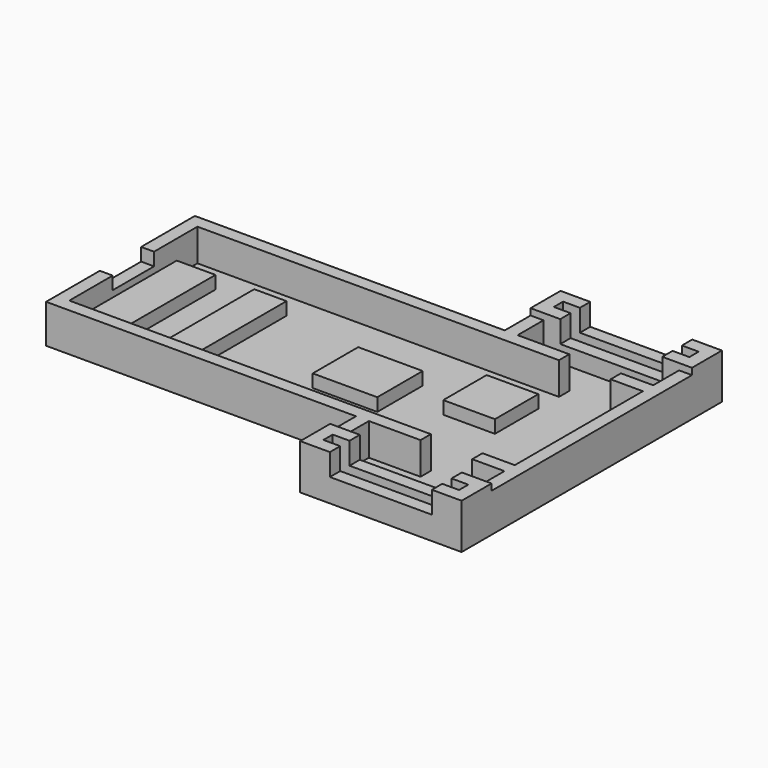
from build123d import *

# Parameters (mm, degrees)
F0_W      = 6
F0_H      = 16.8
F1_DEPTH  = 3
F0_W_2    = 5
F0_W_3    = 10
F0_H_2    = 8.8
F0_W_4    = 8
F0_H_3    = 8.4
F2_DEPTH  = 6
F0_W_5    = 15.8
F0_H_4    = 2
F3_DEPTH  = 3.6
F4_DEPTH  = 1
F7_DEPTH  = 1
F8_DEPTH  = 1
F9_W      = 2
F9_H      = 8
F10_DEPTH = 2


# Not quite as in the source:
# - a feature names something its author has since deleted; it is built from what else it names


with BuildPart() as f1:
    # F0 (on Top) → F1 (new body)
    with BuildSketch(Plane.XY):
        with Locations((3, 12.4)):
            Rectangle(F0_W, F0_H)
    extrude(amount=F1_DEPTH)

    # F0 (on Top) → F2 (join)
    with BuildSketch(Plane.XY):
        Polygon((0, 4), (0, 20.8), (0, 24.8), (56, 24.8), (56, 26.8), (48, 26.8), (48, 31.8), (50.6, 31.8), (50.6, 33.8), (48, 33.8), (48, 35.6), (50.6, 35.6), (50.6, 37.6), (46, 37.6), (46, 26.8), (-2, 26.8), (-2, -2), (46, -2), (46, -12.8), (50.6, -12.8), (50.6, -10.8), (48, -10.8), (48, -9), (50.6, -9), (50.6, -7), (48, -7), (48, -2), (56, -2), (56, 0), (0, 0), align=None)
    extrude(amount=F2_DEPTH)



with BuildPart() as f1b:
    # F0 (on Top) → F1, piece 2 (new body)
    with BuildSketch(Plane.XY):
        with Locations((14.5, 12.4)):
            Rectangle(F0_W_2, F0_H)
    extrude(amount=F1_DEPTH)


with BuildPart() as f1c:
    # F0 (on Top) → F1, piece 3 (new body)
    with BuildSketch(Plane.XY):
        with Locations((36.3, 12.4)):
            Rectangle(F0_W_3, F0_H_2)
    extrude(amount=F1_DEPTH)


with BuildPart() as f1d:
    # F0 (on Top) → F1, piece 4 (new body)
    with BuildSketch(Plane.XY):
        with Locations((52, 16.6)):
            Rectangle(F0_W_4, F0_H_3)
    extrude(amount=F1_DEPTH)


with BuildPart() as f2:
    # F0 (on Top) → F2, piece 2 (new body)
    with BuildSketch(Plane.XY):
        Polygon((66.4, 33.8), (66.4, 31.8), (69, 31.8), (69, 26.8), (64, 26.8), (64, 24.8), (69, 24.8), (69, 0), (64, 0), (64, -2), (69, -2), (69, -7), (66.4, -7), (66.4, -9), (69, -9), (69, -10.8), (66.4, -10.8), (66.4, -12.8), (71, -12.8), (71, 37.6), (66.4, 37.6), (66.4, 35.6), (69, 35.6), (69, 33.8), align=None)
    extrude(amount=F2_DEPTH)


with BuildPart() as f1_1:
    add(f1.part)

    add(f2.part)  # F3 merges F2
    # F0 (on Top) → F3 (join)
    with BuildSketch(Plane.XY):
        with Locations((58.5, 36.6)):
            Rectangle(F0_W_5, F0_H_4)
        with Locations((58.5, 32.8)):
            Rectangle(F0_W_5, F0_H_4)
        with Locations((58.5, -8)):
            Rectangle(F0_W_5, F0_H_4)
        with Locations((58.5, -11.8)):
            Rectangle(F0_W_5, F0_H_4)
    extrude(amount=F3_DEPTH)

    # F0 (on Top) → F4 (join)
    with BuildSketch(Plane.XY):
        Polygon((48, 33.8), (50.6, 33.8), (66.4, 33.8), (69, 33.8), (69, 35.6), (66.4, 35.6), (50.6, 35.6), (48, 35.6), align=None)
        Polygon((66.4, -9), (50.6, -9), (48, -9), (48, -10.8), (50.6, -10.8), (66.4, -10.8), (69, -10.8), (69, -9), align=None)
    extrude(amount=F4_DEPTH)

    # F5 (on face) + F6 (on face) → F7 (join)
    with BuildSketch(Plane.XY.offset(6)):
        Polygon((48, 31.8), (50.6, 31.8), (50.6, 33.8), (48, 33.8), (48, 35.6), (50.6, 35.6), (50.6, 37.6), (46, 37.6), (46, 31.8), align=None)
        Polygon((48, -7), (46, -7), (46, -12.8), (50.6, -12.8), (50.6, -10.8), (48, -10.8), (48, -9), (50.6, -9), (50.6, -7), align=None)
    with BuildSketch(Plane.XY.offset(6)):
        Polygon((66.4, 33.8), (66.4, 31.8), (69, 31.8), (71, 31.8), (71, 37.6), (66.4, 37.6), (66.4, 35.6), (69, 35.6), (69, 33.8), align=None)
        Polygon((71, -12.8), (71, -7), (69, -7), (66.4, -7), (66.4, -9), (69, -9), (69, -10.8), (66.4, -10.8), (66.4, -12.8), align=None)
    extrude(amount=F7_DEPTH)


    add(f1b.part)  # F8 merges F1b

    add(f1c.part)  # F8 merges F1c

    add(f1d.part)  # F8 merges F1d
    # F0 (on Top) → F8 (join)
    with BuildSketch(Plane.XY):
        Polygon((0, 4), (0, 20.8), (0, 24.8), (56, 24.8), (56, 26.8), (48, 26.8), (48, 31.8), (50.6, 31.8), (50.6, 33.8), (48, 33.8), (48, 35.6), (50.6, 35.6), (50.6, 37.6), (46, 37.6), (46, 26.8), (-2, 26.8), (-2, -2), (46, -2), (46, -12.8), (50.6, -12.8), (50.6, -10.8), (48, -10.8), (48, -9), (50.6, -9), (50.6, -7), (48, -7), (48, -2), (56, -2), (56, 0), (0, 0), align=None)
        Polygon((66.4, 33.8), (66.4, 31.8), (69, 31.8), (69, 26.8), (64, 26.8), (64, 24.8), (69, 24.8), (69, 0), (64, 0), (64, -2), (69, -2), (69, -7), (66.4, -7), (66.4, -9), (69, -9), (69, -10.8), (66.4, -10.8), (66.4, -12.8), (71, -12.8), (71, 37.6), (66.4, 37.6), (66.4, 35.6), (69, 35.6), (69, 33.8), align=None)
        with Locations((58.5, 36.6)):
            Rectangle(F0_W_5, F0_H_4)
        with Locations((58.5, -11.8)):
            Rectangle(F0_W_5, F0_H_4)
        Polygon((0, 24.8), (0, 20.8), (6, 20.8), (6, 4), (0, 4), (0, 0), (56, 0), (56, -2), (48, -2), (48, -7), (50.6, -7), (66.4, -7), (69, -7), (69, -2), (64, -2), (64, 0), (69, 0), (69, 24.8), (64, 24.8), (64, 26.8), (69, 26.8), (69, 31.8), (66.4, 31.8), (50.6, 31.8), (48, 31.8), (48, 26.8), (56, 26.8), (56, 24.8), align=None)
        with Locations((14.5, 12.4)):
            Rectangle(F0_W_2, F0_H, mode=Mode.SUBTRACT)
        with Locations((36.3, 12.4)):
            Rectangle(F0_W_3, F0_H_2, mode=Mode.SUBTRACT)
        with Locations((52, 16.6)):
            Rectangle(F0_W_4, F0_H_3, mode=Mode.SUBTRACT)
    extrude(amount=F8_DEPTH)

    # F9 (on face) → F10 (cut)
    with BuildSketch(Plane.XY.offset(6)):
        with Locations((-1, 12.4)):
            Rectangle(F9_W, F9_H)
    extrude(amount=-F10_DEPTH, mode=Mode.SUBTRACT)


solid = f1_1.part
